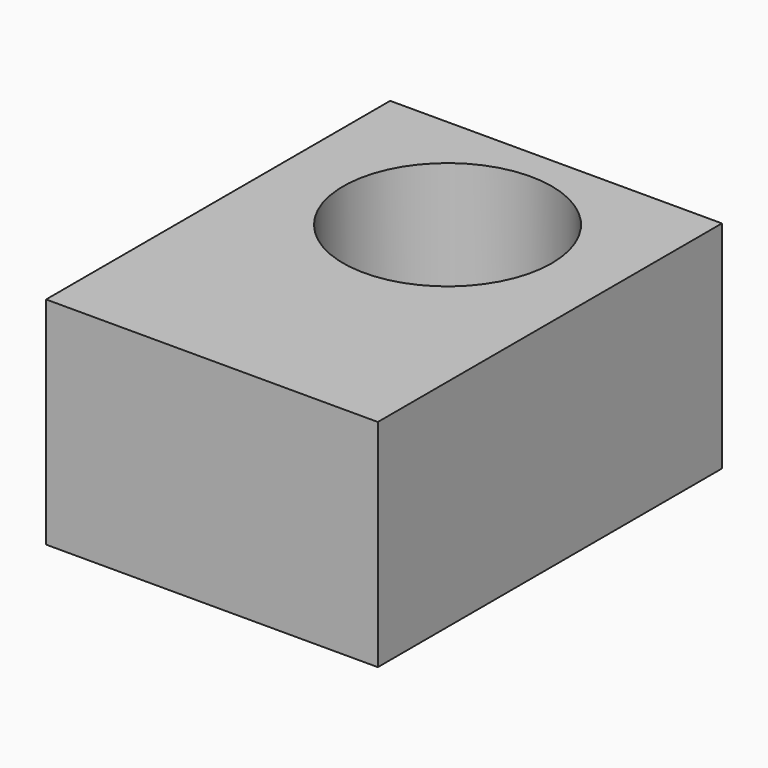
from build123d import *

# Parameters (mm, degrees)
F0_W     = 67.9279565811
F0_H     = 88.0647003651
F1_DEPTH = 44.196
F2_R     = 21.3566300463
F3_DEPTH = 44.197


# Not quite as in the source:
# - a feature of the source that left no trace in its solid (it failed there, or was rolled back) is left out


with BuildPart() as f1:
    # F0 (on Top) → F1 (new body)
    with BuildSketch(Plane.XY):
        Rectangle(F0_W, F0_H)
    extrude(amount=F1_DEPTH)

    # F2 (on face) → F3 (cut, through all)
    with BuildSketch(Plane.XY.offset(44.196)):
        with Locations((0, 16.2552539259)):
            Circle(F2_R)
    extrude(amount=-F3_DEPTH, mode=Mode.SUBTRACT)


solid = f1.part
